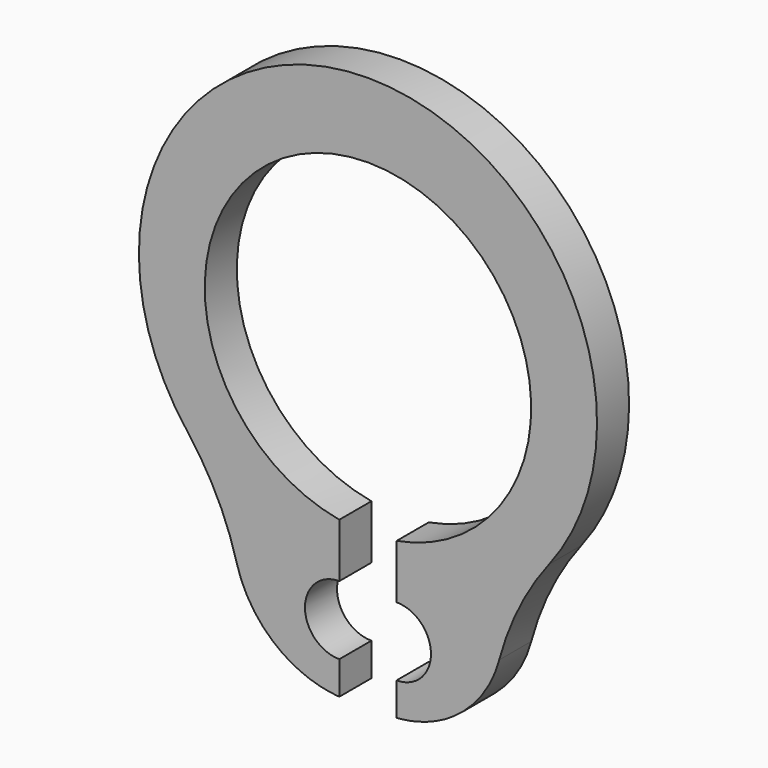
from build123d import *

# Parameters (mm, degrees)
F1_DEPTH    = 0.35
F2_T1_DEPTH = 0.7
F3_R        = 2


# Not quite as in the source:
# - a fillet or chamfer that OpenCascade refuses, or shapes differently, is made with other operations: its cross-section is extruded or revolved along the edge and cut away or added


with BuildPart() as f1:
    # F0 (on Front) → F1 (new body, symmetric)
    with BuildSketch(Plane.XZ):
        with BuildLine():
            ThreePointArc((-0.5, -2.8057975693), (0, 2.85), (0.5, -2.8057975693))
            Line((0.5, -2.8057975693), (0.5, -3.75))
            ThreePointArc((0.5, -3.75), (1.1, -4.35), (0.5, -4.95))
            Line((0.5, -4.95), (0.5, -5.5274315916))
            ThreePointArc((0.5, -5.5274315916), (1.3270959738, -5.3889995617), (2.1238930496, -5.1275314054))
            Line((2.1238930496, -5.1275314054), (1.4775430927, -3.5671045734))
            ThreePointArc((1.4775430927, -3.5671045734), (0, 4.15), (-1.4775430927, -3.5671045734))
            Line((-1.4775430927, -3.5671045734), (-2.1238930496, -5.1275314054))
            ThreePointArc((-2.1238930496, -5.1275314054), (-1.3270959738, -5.3889995617), (-0.5, -5.5274315916))
            Line((-0.5, -5.5274315916), (-0.5, -4.95))
            ThreePointArc((-0.5, -4.95), (-1.1, -4.35), (-0.5, -3.75))
            Line((-0.5, -3.75), (-0.5, -2.8057975693))
        make_face()
    extrude(amount=F1_DEPTH, both=True)

    # F2: fillet of radius 5 on 2 edges, made by hand

    # F2_s2 → F2_t1 (join)
    with BuildSketch(Plane.XZ.offset(-0.35)):
        with BuildLine():
            ThreePointArc((3.163836873, -2.2974754832), (2.4254620947, -3.6322482415), (2.1238930496, -5.1275314054))
            Line((2.1238930496, -5.1275314054), (1.4775430927, -3.5671045734))
            ThreePointArc((1.4775430927, -3.5671045734), (2.4059491896, -3.0455294549), (3.163836873, -2.2974754832))
        make_face()
        with BuildLine():
            ThreePointArc((-2.1238930496, -5.1275314054), (-2.4254620947, -3.6322482415), (-3.163836873, -2.2974754832))
            ThreePointArc((-3.163836873, -2.2974754832), (-2.4059491896, -3.0455294549), (-1.4775430927, -3.5671045734))
            Line((-1.4775430927, -3.5671045734), (-2.1238930496, -5.1275314054))
        make_face()
    extrude(amount=F2_T1_DEPTH)

    # F3
    f3_edges = [f1.edges().sort_by_distance(p)[0] for p in [
        (-2.123893, 0, -5.127531),
        (2.123893, 0, -5.127531),
    ]]
    fillet(f3_edges, radius=F3_R)


solid = f1.part
